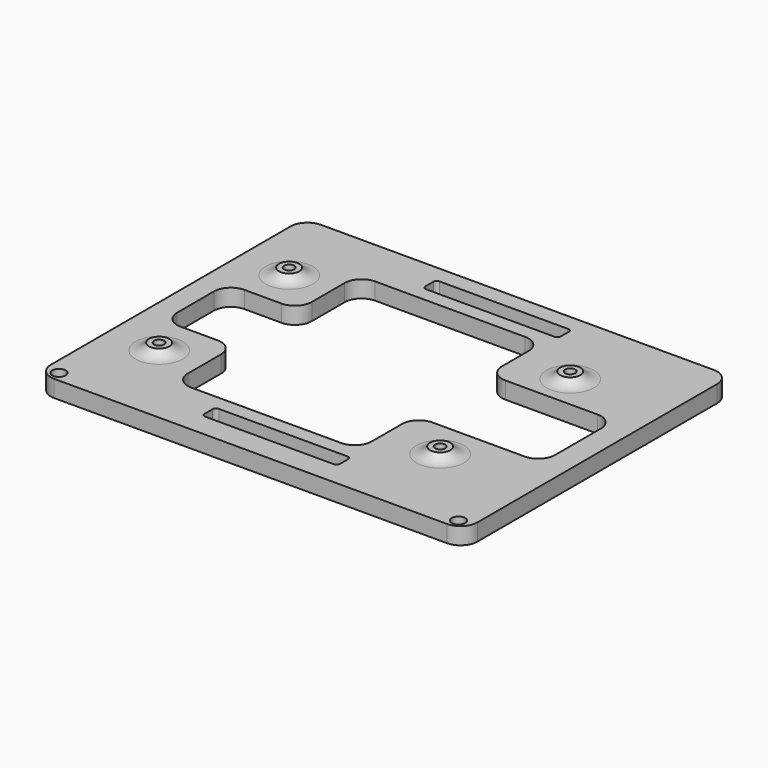
from build123d import *

# Parameters (mm, degrees)
F0_R     = 2
F0_R_2   = 3
F0_R_3   = 1.5
F0_R_4   = 5
F1_DEPTH = 5
F2_R     = 1
F3_R     = 5
F4_DEPTH = 7
F6_W     = 20.916191861
F6_H     = 23.5347189009
F6_W_2   = 37.2305270284
F6_H_2   = 26.8968194723
F7_DEPTH = 25
F8_R     = 5


# Not quite as in the source:
# - a fillet or chamfer that OpenCascade refuses, or shapes differently, is made with other operations: its cross-section is extruded or revolved along the edge and cut away or added


with BuildPart() as f1:
    # F0 (on Top) → F1 (new body)
    with BuildSketch(Plane.XY):
        Polygon((-49.7560231508, 7), (-49.7560231508, 0), (76.2439768492, 0), (76.2439768492, 7), (33.2439768492, 7), (-6.7560231508, 7), align=None)
        with Locations((-45.7560231508, 3)):
            Circle(F0_R, mode=Mode.SUBTRACT)
        with Locations((72.2439768492, 3)):
            Circle(F0_R, mode=Mode.SUBTRACT)
        Polygon((-49.7560231508, 93.5), (-49.7560231508, 7), (-6.7560231508, 7), (-6.7560231508, 12), (33.2439768492, 12), (33.2439768492, 7), (76.2439768492, 7), (76.2439768492, 93.5), (33.2439768492, 93.5), (33.2439768492, 88.5), (-6.7560231508, 88.5), (-6.7560231508, 93.5), align=None)
        with Locations((-34.7560231508, 26.25)):
            Circle(F0_R_2, mode=Mode.SUBTRACT)
        with Locations((3.2439768492, 40.25)):
            Circle(F0_R_3, mode=Mode.SUBTRACT)
        with Locations((23.2439768492, 40.25)):
            Circle(F0_R_3, mode=Mode.SUBTRACT)
        with Locations((48.2439768492, 26.25)):
            Circle(F0_R_2, mode=Mode.SUBTRACT)
        with Locations((3.2439768492, 60.25)):
            Circle(F0_R_3, mode=Mode.SUBTRACT)
        with Locations((-34.7560231508, 74.25)):
            Circle(F0_R_2, mode=Mode.SUBTRACT)
        with Locations((13.2439768492, 50.25)):
            Circle(F0_R_4, mode=Mode.SUBTRACT)
        with Locations((23.2439768492, 60.25)):
            Circle(F0_R_3, mode=Mode.SUBTRACT)
        with Locations((48.2439768492, 74.25)):
            Circle(F0_R_2, mode=Mode.SUBTRACT)
        Polygon((-49.7560231508, 98.5), (-49.7560231508, 93.5), (-6.7560231508, 93.5), (33.2439768492, 93.5), (76.2439768492, 93.5), (76.2439768492, 98.5), align=None)
        with Locations((-34.7560231508, 26.25)):
            Circle(F0_R_2)
        with Locations((-34.7560231508, 26.25)):
            Circle(F0_R_3, mode=Mode.SUBTRACT)
        with Locations((-34.7560231508, 74.25)):
            Circle(F0_R_2)
        with Locations((-34.7560231508, 74.25)):
            Circle(F0_R_3, mode=Mode.SUBTRACT)
        with Locations((48.2439768492, 26.25)):
            Circle(F0_R_2)
        with Locations((48.2439768492, 26.25)):
            Circle(F0_R_3, mode=Mode.SUBTRACT)
        with Locations((48.2439768492, 74.25)):
            Circle(F0_R_2)
        with Locations((48.2439768492, 74.25)):
            Circle(F0_R_3, mode=Mode.SUBTRACT)
        with Locations((13.2439768492, 50.25)):
            Circle(F0_R_4)
        with Locations((3.2439768492, 60.25)):
            Circle(F0_R_3)
        with Locations((3.2439768492, 40.25)):
            Circle(F0_R_3)
        with Locations((23.2439768492, 40.25)):
            Circle(F0_R_3)
        with Locations((23.2439768492, 60.25)):
            Circle(F0_R_3)
    extrude(amount=F1_DEPTH)

    # F2
    f2_edges = [f1.edges().sort_by_distance(p)[0] for p in [
        (-6.756023, 12, 2.5),
        (33.243977, 12, 2.5),
        (-6.756023, 7, 2.5),
        (33.243977, 7, 2.5),
        (-6.756023, 88.5, 2.5),
        (-6.756023, 93.5, 2.5),
        (33.243977, 93.5, 2.5),
        (33.243977, 88.5, 2.5),
    ]]
    fillet(f2_edges, radius=F2_R)

    # F3
    f3_edges = [f1.edges().sort_by_distance(p)[0] for p in [
        (-49.756023, 0, 2.5),
        (76.243977, 0, 2.5),
        (76.243977, 98.5, 2.5),
        (-49.756023, 98.5, 2.5),
    ]]
    fillet(f3_edges, radius=F3_R)

    # F0 (on Top) → F4 (join)
    with BuildSketch(Plane.XY):
        with Locations((-34.7560231508, 74.25)):
            Circle(F0_R_2)
        with Locations((-34.7560231508, 74.25)):
            Circle(F0_R_3, mode=Mode.SUBTRACT)
        with Locations((-34.7560231508, 26.25)):
            Circle(F0_R_2)
        with Locations((-34.7560231508, 26.25)):
            Circle(F0_R_3, mode=Mode.SUBTRACT)
        with Locations((48.2439768492, 74.25)):
            Circle(F0_R_2)
        with Locations((48.2439768492, 74.25)):
            Circle(F0_R_3, mode=Mode.SUBTRACT)
        with Locations((48.2439768492, 26.25)):
            Circle(F0_R_2)
        with Locations((48.2439768492, 26.25)):
            Circle(F0_R_3, mode=Mode.SUBTRACT)
    extrude(amount=F4_DEPTH)

    # F5: fillet of radius 5 on 4 edges, made by hand

    # F5_s1 → F5_t2 (revolve)
    with BuildSketch(Plane.XZ.offset(-74.25)):
        with BuildLine():
            ThreePointArc((-27.7560231508, 5), (-29.9920911283, 5.527864045), (-31.7560231508, 7))
            Line((-31.7560231508, 7), (-31.7560231508, 5))
            Line((-31.7560231508, 5), (-27.7560231508, 5))
        make_face()
    revolve(axis=Axis((-34.7560231508, 74.25, 5), (0, 0, -1)))

    # F5_s3 → F5_t4 (revolve)
    with BuildSketch(Plane.XZ.offset(-26.25)):
        with BuildLine():
            ThreePointArc((-27.7560231508, 5), (-29.9920911283, 5.527864045), (-31.7560231508, 7))
            Line((-31.7560231508, 7), (-31.7560231508, 5))
            Line((-31.7560231508, 5), (-27.7560231508, 5))
        make_face()
    revolve(axis=Axis((-34.7560231508, 26.25, 5), (0, 0, -1)))

    # F5_s5 → F5_t6 (revolve)
    with BuildSketch(Plane.XZ.offset(-26.25)):
        with BuildLine():
            ThreePointArc((55.2439768492, 5), (53.0079088717, 5.527864045), (51.2439768492, 7))
            Line((51.2439768492, 7), (51.2439768492, 5))
            Line((51.2439768492, 5), (55.2439768492, 5))
        make_face()
    revolve(axis=Axis((48.2439768492, 26.25, 5), (0, 0, -1)))

    # F5_s7 → F5_t8 (revolve)
    with BuildSketch(Plane.XZ.offset(-74.25)):
        with BuildLine():
            ThreePointArc((51.2439768492, 7), (53.0079088717, 5.527864045), (55.2439768492, 5))
            Line((55.2439768492, 5), (51.2439768492, 5))
            Line((51.2439768492, 5), (51.2439768492, 7))
        make_face()
    revolve(axis=Axis((48.2439768492, 74.25, 5), (0, 0, -1)))

    # F6 (on face) → F7 (cut)
    with BuildSketch(Plane.XY.offset(5)):
        Polygon((31.9697726518, 84.2200964689), (-22.3512705415, 84.2200964689), (-22.3512705415, 62.1007867157), (-22.3512705415, 38.5660678148), (-22.3512705415, 16.3328051567), (31.9697726518, 16.3328051567), (31.9697726518, 37.4815165997), (31.9697726518, 64.378336072), align=None)
        with Locations((-32.8093664721, 50.3334272653)):
            Rectangle(F6_W, F6_H)
        with Locations((50.585036166, 50.9299263358)):
            Rectangle(F6_W_2, F6_H_2)
    extrude(amount=-F7_DEPTH, mode=Mode.SUBTRACT)

    # F8
    f8_edges = [f1.edges().sort_by_distance(p)[0] for p in [
        (-22.351271, 62.100787, 2.5),
        (31.969773, 64.378336, 2.5),
        (31.969773, 37.481517, 2.5),
        (-22.351271, 38.566068, 2.5),
        (-43.267462, 38.566068, 2.5),
        (-43.267462, 62.100787, 2.5),
        (-22.351271, 84.220096, 2.5),
        (31.969773, 84.220096, 2.5),
        (69.2003, 64.378336, 2.5),
        (69.2003, 37.481517, 2.5),
        (31.969773, 16.332805, 2.5),
        (-22.351271, 16.332805, 2.5),
    ]]
    fillet(f8_edges, radius=F8_R)


solid = f1.part
